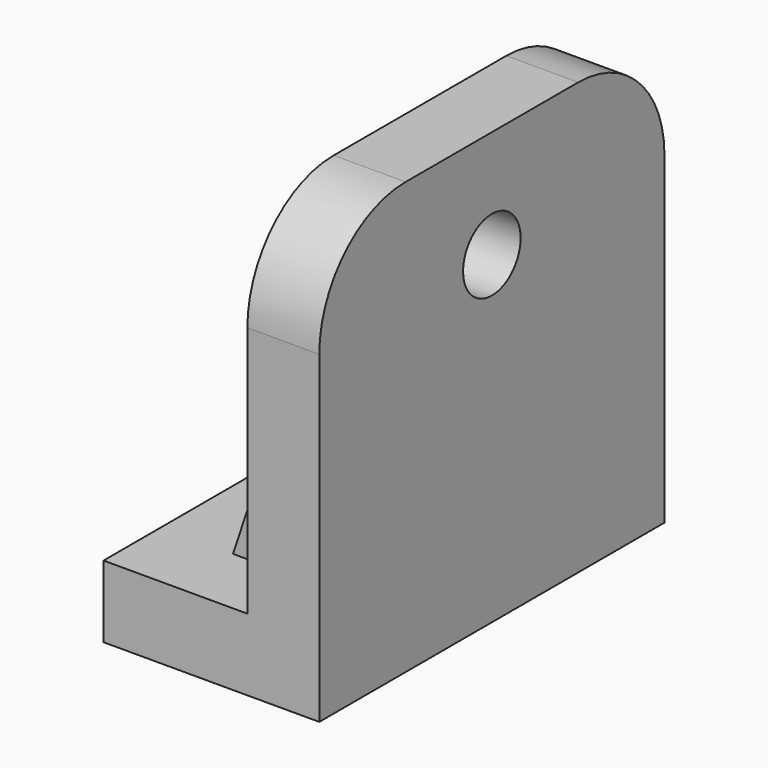
from build123d import *

# Parameters (mm, degrees)
F1_DEPTH  = 76.2
F2_R      = 12.7
F3_DEPTH  = 76.201
F5_DEPTH  = 25.401
F6_R      = 38.1
F7_R      = 19.05
F7_R_2    = 12.7
F8_DEPTH  = 6.35
F11_DEPTH = 6.35


# Not quite as in the source:
# - a pattern or mirror of a feature is missing from the dataset's text; its kind, count and spacing are read off the source's solid


with BuildPart() as f1:
    # F0 (on Front) → F1 (new body, symmetric)
    with BuildSketch(Plane.XZ):
        Polygon((-76.2, 0), (0, 0), (0, 152.4), (-25.4, 152.4), (-25.4, 25.4), (-76.2, 25.4), align=None)
    extrude(amount=F1_DEPTH, both=True)

    # F2 (on face) → F3 (cut, through all)
    with BuildSketch(Plane.YZ):
        with Locations((0, 114.3)):
            Circle(F2_R)
    extrude(amount=-F3_DEPTH, mode=Mode.SUBTRACT)

    # F4 (on face) → F5 (cut, through all)
    with BuildSketch(Plane.XY.offset(25.4)):
        with BuildLine():
            Line((-63.5, 12.7), (-76.2, 12.7))
            Line((-76.2, 12.7), (-76.2, -12.7))
            Line((-76.2, -12.7), (-63.5, -12.7))
            ThreePointArc((-63.5, -12.7), (-50.8, 0), (-63.5, 12.7))
        make_face()
    extrude(amount=-F5_DEPTH, mode=Mode.SUBTRACT)

    # F6
    f6_edges = [f1.edges().sort_by_distance(p)[0] for p in [
        (-12.7, -76.2, 152.4),
        (-12.7, 76.2, 152.4),
    ]]
    fillet(f6_edges, radius=F6_R)

    # F7 (on face) → F8 (cut)
    with BuildSketch(Plane(origin=(-25.4, 0, 0), x_dir=(0, -1, 0), z_dir=(-1, 0, 0))):
        with Locations((0, 114.3)):
            Circle(F7_R)
        with Locations((0, 114.3)):
            Circle(F7_R_2, mode=Mode.SUBTRACT)
    extrude(amount=-F8_DEPTH, mode=Mode.SUBTRACT)

    # F10 (on offset) → F11 (join, symmetric)
    with BuildSketch(Plane.XZ.offset(44.45)):
        Polygon((-50.8, 25.4), (-25.4, 25.4), (-25.4, 101.6), align=None)
    f11 = extrude(amount=F11_DEPTH, both=True)

    # F11_copies: F11 across plane
    add(f11.mirror(Plane.ZX))


solid = f1.part
